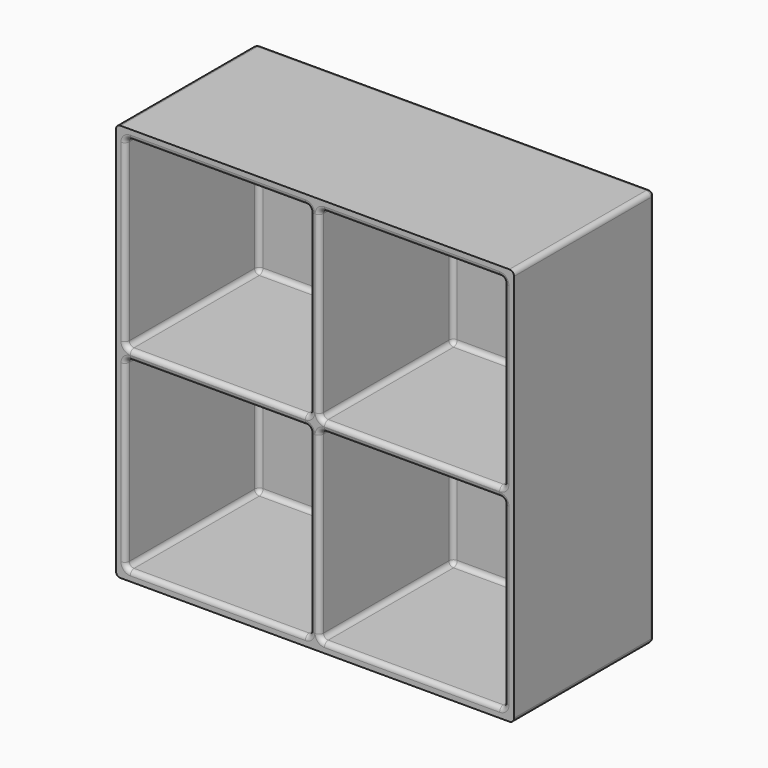
from build123d import *

# Parameters (mm, degrees)
F0_W     = 129.54
F0_H     = 129.54
F1_DEPTH = 57.15
F2_T     = -3.175
F3_R     = 1.524
F4_R     = 1.524
F5_W     = 3.175
F5_H     = 1.524
F5_H_2   = 120.142
F6_DEPTH = 53.975
F7_W     = 60.0075
F7_H     = 3.175
F8_DEPTH = 53.975
F9_R     = 1.524


with BuildPart() as f1:
    # F0 (on Front) → F1 (new body)
    with BuildSketch(Plane.XZ):
        with Locations((64.77, 64.77)):
            Rectangle(F0_W, F0_H)
    extrude(amount=-F1_DEPTH)

    # F2
    f2_openings = [f1.faces().sort_by_distance(p)[0] for p in [
        (64.77, 0, 64.77),
    ]]
    offset(amount=F2_T, openings=f2_openings)

    # F3
    f3_edges = [f1.edges().sort_by_distance(p)[0] for p in [
        (3.175, 26.9875, 126.365),
        (64.77, 53.975, 126.365),
        (3.175, 53.975, 64.77),
        (3.175, 26.9875, 3.175),
        (64.77, 53.975, 3.175),
        (126.365, 53.975, 64.77),
        (126.365, 26.9875, 126.365),
        (126.365, 26.9875, 3.175),
    ]]
    fillet(f3_edges, radius=F3_R)

    # F4
    f4_edges = [f1.edges().sort_by_distance(p)[0] for p in [
        (129.54, 28.575, 0),
        (64.77, 57.15, 0),
        (129.54, 57.15, 64.77),
        (129.54, 28.575, 129.54),
        (64.77, 57.15, 129.54),
        (0, 28.575, 129.54),
        (0, 57.15, 64.77),
        (0, 28.575, 0),
    ]]
    fillet(f4_edges, radius=F4_R)

    # F5 (on face) → F6 (join)
    with BuildSketch(Plane.XZ.offset(-53.975)):
        with Locations((64.77, 125.603)):
            Rectangle(F5_W, F5_H)
        with Locations((64.77, 64.77)):
            Rectangle(F5_W, F5_H_2)
        with Locations((64.77, 3.937)):
            Rectangle(F5_W, F5_H)
    extrude(amount=F6_DEPTH)

    # F7 (on face) → F8 (join)
    with BuildSketch(Plane.XZ):
        with BuildLine():
            ThreePointArc((1.524, 129.54), (0.4463692655, 129.0936307345), (0, 128.016))
            Line((0, 128.016), (0, 1.524))
            ThreePointArc((0, 1.524), (0.4463692655, 0.4463692655), (1.524, 0))
            Line((1.524, 0), (128.016, 0))
            ThreePointArc((128.016, 0), (129.0936307345, 0.4463692655), (129.54, 1.524))
            Line((129.54, 1.524), (129.54, 128.016))
            ThreePointArc((129.54, 128.016), (129.0936307345, 129.0936307345), (128.016, 129.54))
            Line((128.016, 129.54), (1.524, 129.54))
        make_face()
        with BuildLine():
            Line((3.175, 4.699), (3.175, 63.1825))
            Line((3.175, 63.1825), (3.175, 66.3575))
            Line((3.175, 66.3575), (3.175, 124.841))
            ThreePointArc((3.175, 124.841), (3.6213692655, 125.9186307345), (4.699, 126.365))
            Line((4.699, 126.365), (63.1825, 126.365))
            Line((63.1825, 126.365), (63.1825, 66.3575))
            Line((63.1825, 66.3575), (66.3575, 66.3575))
            Line((66.3575, 66.3575), (66.3575, 126.365))
            Line((66.3575, 126.365), (124.841, 126.365))
            ThreePointArc((124.841, 126.365), (125.9186307345, 125.9186307345), (126.365, 124.841))
            Line((126.365, 124.841), (126.365, 66.3575))
            Line((126.365, 66.3575), (126.365, 63.1825))
            Line((126.365, 63.1825), (126.365, 4.699))
            ThreePointArc((126.365, 4.699), (125.9186307345, 3.6213692655), (124.841, 3.175))
            Line((124.841, 3.175), (66.3575, 3.175))
            Line((66.3575, 3.175), (66.3575, 63.1825))
            Line((66.3575, 63.1825), (63.1825, 63.1825))
            Line((63.1825, 63.1825), (63.1825, 3.175))
            Line((63.1825, 3.175), (4.699, 3.175))
            ThreePointArc((4.699, 3.175), (3.6213692655, 3.6213692655), (3.175, 4.699))
        make_face(mode=Mode.SUBTRACT)
        with Locations((33.17875, 64.77)):
            Rectangle(F7_W, F7_H)
        with Locations((96.36125, 64.77)):
            Rectangle(F7_W, F7_H)
    extrude(amount=-F8_DEPTH)

    # F9
    f9_edges = [f1.edges().sort_by_distance(p)[0] for p in [
        (66.3575, 53.975, 95.59925),
        (66.3575, 53.528631, 125.918631),
        (66.3575, 26.2255, 126.365),
        (66.3575, 0, 96.36125),
        (66.3575, 26.9875, 66.3575),
        (96.36125, 0, 66.3575),
        (95.59925, 53.975, 66.3575),
        (125.918631, 53.528631, 66.3575),
        (126.365, 26.2255, 66.3575),
        (126.365, 0, 95.59925),
        (126.365, 26.2255, 124.841),
        (126.365, 52.451, 95.59925),
        (126.365, 0, 33.94075),
        (126.365, 26.2255, 63.1825),
        (126.365, 52.451, 33.94075),
        (126.365, 26.2255, 4.699),
        (96.36125, 0, 63.1825),
        (125.918631, 53.528631, 63.1825),
        (95.59925, 53.975, 63.1825),
        (66.3575, 26.9875, 63.1825),
        (66.3575, 53.975, 33.94075),
        (66.3575, 0, 33.17875),
        (66.3575, 26.2255, 3.175),
        (66.3575, 53.528631, 3.621369),
        (95.59925, 0, 3.175),
        (124.841, 26.2255, 3.175),
        (95.59925, 52.451, 3.175),
        (33.94075, 0, 3.175),
        (63.1825, 26.2255, 3.175),
        (33.94075, 52.451, 3.175),
        (4.699, 26.2255, 3.175),
        (3.175, 0, 33.94075),
        (3.175, 26.2255, 4.699),
        (3.175, 52.451, 33.94075),
        (3.175, 26.2255, 63.1825),
        (33.17875, 0, 63.1825),
        (63.1825, 26.9875, 63.1825),
        (33.94075, 53.975, 63.1825),
        (3.621369, 53.528631, 63.1825),
        (63.1825, 53.975, 33.94075),
        (63.1825, 53.528631, 3.621369),
        (63.1825, 0, 33.17875),
        (95.59925, 0, 126.365),
        (95.59925, 52.451, 126.365),
        (124.841, 26.2255, 126.365),
        (33.94075, 0, 126.365),
        (4.699, 26.2255, 126.365),
        (33.94075, 52.451, 126.365),
        (63.1825, 26.2255, 126.365),
        (63.1825, 53.975, 95.59925),
        (63.1825, 26.9875, 66.3575),
        (63.1825, 0, 96.36125),
        (63.1825, 53.528631, 125.918631),
        (33.17875, 0, 66.3575),
        (3.175, 26.2255, 66.3575),
        (3.621369, 53.528631, 66.3575),
        (33.94075, 53.975, 66.3575),
        (3.175, 0, 95.59925),
        (3.175, 52.451, 95.59925),
        (3.175, 26.2255, 124.841),
        (3.621369, 0, 125.918631),
        (3.621369, 0, 3.621369),
        (125.918631, 0, 3.621369),
        (125.918631, 0, 125.918631),
    ]]
    fillet(f9_edges, radius=F9_R)


solid = f1.part
